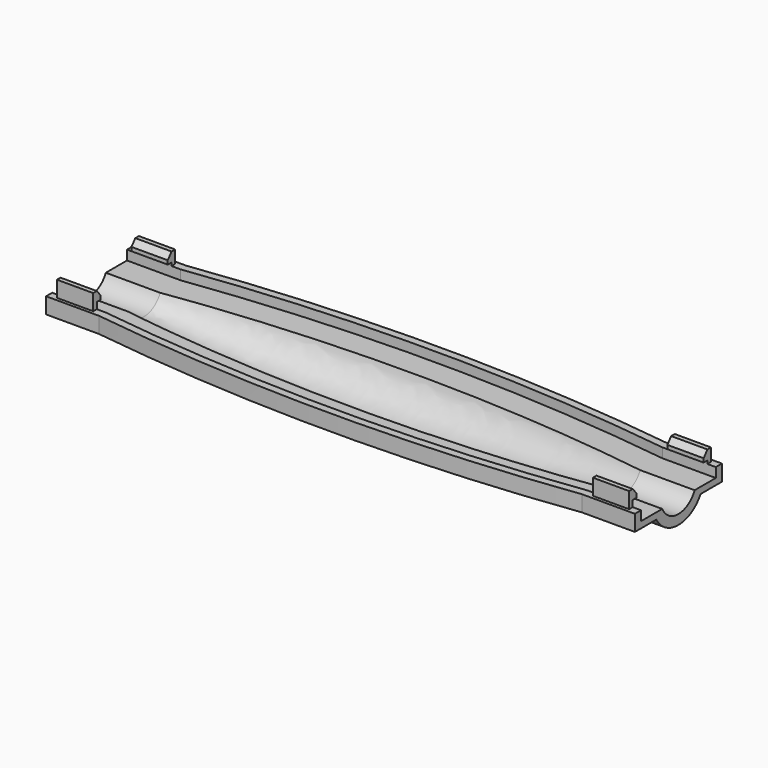
from build123d import *

# Parameters (mm, degrees)
F1_ANGLE  = 180
F3_DEPTH  = 5
F5_DEPTH  = 5
F7_DEPTH  = 3
F9_DEPTH  = 17
F11_DEPTH = 17
F13_DEPTH = 3
F15_DEPTH = 17
F17_DEPTH = 17
F19_DEPTH = 3
F21_DEPTH = 3
F22_W     = 11.3347762211
F22_H     = 1.4
F23_DEPTH = 4
F24_W     = 11.3347762211
F24_H     = 2.4
F25_DEPTH = 5
F27_DEPTH = 11.3347762211
F28_W     = 11.3347762211
F28_H     = 5
F29_DEPTH = 1
F31_DEPTH = 11.3347762211
F32_W     = 11.3347762211
F32_H     = 5
F33_DEPTH = 1
F35_DEPTH = 11.3347762211
F37_DEPTH = 11.3347762211


with BuildPart() as f1:
    # F0 (on Top) → F1 (revolve)
    with BuildSketch(Plane.XY):
        with BuildLine():
            ThreePointArc((-75, 7), (0, 12), (75, 7))
            Line((75, 7), (92, 7))
            Line((92, 7), (92, 10))
            Line((92, 10), (75, 10))
            ThreePointArc((75, 10), (0, 15), (-75, 10))
            Line((-75, 10), (-92, 10))
            Line((-92, 10), (-92, 7))
            Line((-92, 7), (-75, 7))
        make_face()
    revolve(axis=Axis((-37.5, 0, 0), (-1, 0, 0)), revolution_arc=F1_ANGLE)

    # F2 (on face) → F3 (join)
    with BuildSketch(Plane.XY):
        with BuildLine():
            Line((-75, 10), (-92, 10))
            Line((-92, 10), (-92, 7))
            Line((-92, 7), (-75, 7))
            ThreePointArc((-75, 7), (0, 12), (75, 7))
            Line((75, 7), (92, 7))
            Line((92, 7), (92, 10))
            Line((92, 10), (75, 10))
            ThreePointArc((75, 10), (0, 15), (-75, 10))
        make_face()
        with BuildLine():
            Line((-75.4652237789, 17), (-92, 17))
            Line((-92, 17), (-92, 10))
            Line((-92, 10), (-75, 10))
            ThreePointArc((-75, 10), (0, 15), (75, 10))
            Line((75, 10), (92, 10))
            Line((92, 10), (92, 17))
            Line((92, 17), (75.4652237789, 17))
            ThreePointArc((75.4652237789, 17), (0, 22), (-75.4652237789, 17))
        make_face()
    extrude(amount=-F3_DEPTH)

    # F4 (on face) → F5 (join)
    with BuildSketch(Plane.XY):
        with BuildLine():
            Line((-92, -7), (-92, -10))
            Line((-92, -10), (-75, -10))
            ThreePointArc((-75, -10), (0, -15), (75, -10))
            Line((75, -10), (92, -10))
            Line((92, -10), (92, -7))
            Line((92, -7), (75, -7))
            ThreePointArc((75, -7), (0, -12), (-75, -7))
            Line((-75, -7), (-92, -7))
        make_face()
        with BuildLine():
            Line((-92, -10), (-92, -17))
            Line((-92, -17), (-75.4652237789, -17))
            ThreePointArc((-75.4652237789, -17), (0, -22), (75.4652237789, -17))
            Line((75.4652237789, -17), (92, -17))
            Line((92, -17), (92, -10))
            Line((92, -10), (75, -10))
            ThreePointArc((75, -10), (0, -15), (-75, -10))
            Line((-75, -10), (-92, -10))
        make_face()
    extrude(amount=-F5_DEPTH)

    # F6 (on face) → F7 (cut)
    with BuildSketch(Plane.XY):
        with BuildLine():
            Line((-75.3060422543, 14.6), (-92, 14.6))
            Line((-92, 14.6), (-92, 7))
            Line((-92, 7), (-75, 7))
            Line((-75, 7), (-75, 8.8160197075))
            ThreePointArc((-75, 8.8160197075), (0, 13.8), (75, 8.8160197075))
            Line((75, 8.8160197075), (75, 7))
            Line((75, 7), (92, 7))
            Line((92, 7), (92, 14.6))
            Line((92, 14.6), (75.3060422543, 14.6))
            ThreePointArc((75.3060422543, 14.6), (0, 19.6), (-75.3060422543, 14.6))
        make_face()
        with BuildLine():
            Line((-75, 8.8160197075), (-75, 7))
            ThreePointArc((-75, 7), (0, 12), (75, 7))
            Line((75, 7), (75, 8.8160197075))
            ThreePointArc((75, 8.8160197075), (0, 13.8), (-75, 8.8160197075))
        make_face()
    extrude(amount=-F7_DEPTH, mode=Mode.SUBTRACT)

    # F8 (on face) → F9 (cut)
    with BuildSketch(Plane(origin=(-92, 0, 0), x_dir=(0, -1, 0), z_dir=(-1, 0, 0))):
        with BuildLine():
            Line((-7, 0), (-7, -3))
            Line((-7, -3), (-6.3245553203, -3))
            ThreePointArc((-6.3245553203, -3), (-6.8290514437, -1.5375488216), (-7, 0))
        make_face()
    extrude(amount=-F9_DEPTH, mode=Mode.SUBTRACT)

    # F10 (on face) → F11 (cut)
    with BuildSketch(Plane.YZ.offset(92)):
        with BuildLine():
            Line((6.3245553203, -3), (7, -3))
            Line((7, -3), (7, 0))
            ThreePointArc((7, 0), (6.8290514437, -1.5375488216), (6.3245553203, -3))
        make_face()
    extrude(amount=-F11_DEPTH, mode=Mode.SUBTRACT)

    # F12 (on face) → F13 (cut)
    with BuildSketch(Plane.XY):
        with BuildLine():
            Line((-92, -7), (-92, -8.8))
            Line((-92, -8.8), (-75.1199041533, -8.8))
            ThreePointArc((-75.1199041533, -8.8), (-75.059952504, -8.8080130526), (-75, -8.8160197075))
            Line((-75, -8.8160197075), (-75, -7))
            Line((-75, -7), (-92, -7))
        make_face()
        with BuildLine():
            Line((-92, -8.8), (-92, -14.6))
            Line((-92, -14.6), (-75.3060422543, -14.6))
            ThreePointArc((-75.3060422543, -14.6), (0, -19.6), (75.3060422543, -14.6))
            Line((75.3060422543, -14.6), (92, -14.6))
            Line((92, -14.6), (92, -8.8))
            Line((92, -8.8), (75.1199041533, -8.8))
            ThreePointArc((75.1199041533, -8.8), (75.059952504, -8.8080130526), (75, -8.8160197075))
            ThreePointArc((75, -8.8160197075), (0, -13.8), (-75, -8.8160197075))
            ThreePointArc((-75, -8.8160197075), (-75.059952504, -8.8080130526), (-75.1199041533, -8.8))
            Line((-75.1199041533, -8.8), (-92, -8.8))
        make_face()
        with BuildLine():
            Line((75.1199041533, -8.8), (92, -8.8))
            Line((92, -8.8), (92, -7))
            Line((92, -7), (75, -7))
            Line((75, -7), (75, -8.8160197075))
            ThreePointArc((75, -8.8160197075), (75.059952504, -8.8080130526), (75.1199041533, -8.8))
        make_face()
    extrude(amount=-F13_DEPTH, mode=Mode.SUBTRACT)

    # F14 (on face) → F15 (cut)
    with BuildSketch(Plane(origin=(-92, 0, 0), x_dir=(0, -1, 0), z_dir=(-1, 0, 0))):
        with BuildLine():
            Line((6.3245553203, -3), (7, -3))
            Line((7, -3), (7, 0))
            ThreePointArc((7, 0), (6.8290514437, -1.5375488216), (6.3245553203, -3))
        make_face()
    extrude(amount=-F15_DEPTH, mode=Mode.SUBTRACT)

    # F16 (on face) → F17 (cut)
    with BuildSketch(Plane.YZ.offset(92)):
        with BuildLine():
            Line((-7, 0), (-7, -3))
            Line((-7, -3), (-6.3245553203, -3))
            ThreePointArc((-6.3245553203, -3), (-6.8290514437, -1.5375488216), (-7, 0))
        make_face()
    extrude(amount=-F17_DEPTH, mode=Mode.SUBTRACT)

    # F18 (on face) → F19 (cut)
    with BuildSketch(Plane.XY):
        with BuildLine():
            ThreePointArc((75, 7), (0, 12), (-75, 7))
            Line((-75, 7), (-75, 5.4070060141))
            Line((-75, 5.4070060141), (75, 5.4070060141))
            Line((75, 5.4070060141), (75, 7))
        make_face()
    extrude(amount=-F19_DEPTH, mode=Mode.SUBTRACT)

    # F20 (on face) → F21 (cut)
    with BuildSketch(Plane.XY):
        with BuildLine():
            Line((-75, -5.2931243554), (-75, -7))
            ThreePointArc((-75, -7), (0, -12), (75, -7))
            Line((75, -7), (75, -5.2931243554))
            Line((75, -5.2931243554), (-75, -5.2931243554))
        make_face()
        with BuildLine():
            Line((-75, -7), (-75, -8.8160197075))
            ThreePointArc((-75, -8.8160197075), (0, -13.8), (75, -8.8160197075))
            Line((75, -8.8160197075), (75, -7))
            ThreePointArc((75, -7), (0, -12), (-75, -7))
        make_face()
    extrude(amount=-F21_DEPTH, mode=Mode.SUBTRACT)

    # F22 (on face) → F23 (join)
    with BuildSketch(Plane.XY):
        with Locations((83.7326118895, 15.3)):
            Rectangle(F22_W, F22_H)
        with Locations((-83.7326118895, 15.3)):
            Rectangle(F22_W, F22_H)
    extrude(amount=F23_DEPTH)

    # F24 (on face) → F25 (join)
    with BuildSketch(Plane.XY):
        with Locations((83.7326118895, -15.8)):
            Rectangle(F24_W, F24_H)
        with Locations((-83.7326118895, -15.8)):
            Rectangle(F24_W, F24_H)
    extrude(amount=F25_DEPTH)

    # F26 (on face) → F27 (join, through all)
    with BuildSketch(Plane(origin=(-89.4, 0, 0), x_dir=(0, -1, 0), z_dir=(-1, 0, 0))):
        Polygon((13.1, 3.2), (13.1, 2), (14.6, 2), (14.6, 5), align=None)
    extrude(amount=-F27_DEPTH)

    # F28 (on face) → F29 (cut)
    with BuildSketch(Plane.XZ.offset(17)):
        with Locations((-83.7326118895, 2.5)):
            Rectangle(F28_W, F28_H)
    extrude(amount=-F29_DEPTH, mode=Mode.SUBTRACT)

    # F30 (on face) → F31 (join, through all)
    with BuildSketch(Plane.YZ.offset(89.4)):
        Polygon((-14.6, 5), (-14.6, 2), (-13.1, 2), (-13.1, 3.2), align=None)
    extrude(amount=-F31_DEPTH)

    # F32 (on face) → F33 (cut)
    with BuildSketch(Plane.XZ.offset(17)):
        with Locations((83.7326118895, 2.5)):
            Rectangle(F32_W, F32_H)
    extrude(amount=-F33_DEPTH, mode=Mode.SUBTRACT)

    # F34 (on face) → F35 (join, through all)
    with BuildSketch(Plane.YZ.offset(89.4)):
        Polygon((13.1, 1), (14.6, 1), (14.6, 4), (13.1, 2.2), align=None)
    extrude(amount=-F35_DEPTH)

    # F36 (on face) → F37 (join, through all)
    with BuildSketch(Plane(origin=(-89.4, 0, 0), x_dir=(0, -1, 0), z_dir=(-1, 0, 0))):
        Polygon((-14.6, 4), (-14.6, 1), (-13.1, 1), (-13.1, 2.2), align=None)
    extrude(amount=-F37_DEPTH)


solid = f1.part
